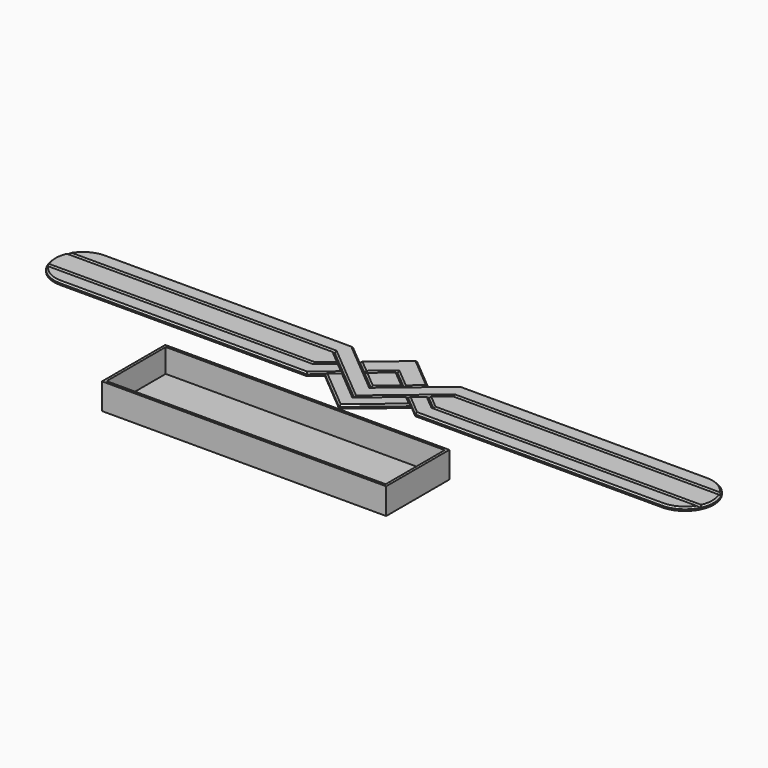
from build123d import *

# Parameters (mm, degrees)
F1_DEPTH  = 2
F3_DEPTH  = 2
F5_DEPTH  = 2
F7_DEPTH  = 2
F9_DEPTH  = 1
F12_DEPTH = 2
F13_SIZE  = 0.99999
F14_W     = 180
F14_H     = 50
F15_DEPTH = 1.6
F16_W     = 180
F16_H     = 50
F16_W_2   = 176.8
F16_H_2   = 46.8
F17_DEPTH = 15


# Not quite as in the source:
# - a fillet or chamfer is up to 0.001 mm smaller than in the source, because OpenCascade refuses the exact size


with BuildPart() as f1:
    # F0 (on Top) → F1 (new body)
    with BuildSketch(Plane.XY):
        Polygon((37.9150851114, 8), (28.3810563706, 0), (37.9150851114, -8), (210, -8), (210, 0), (210, 8), align=None)
    extrude(amount=F1_DEPTH)


with BuildPart() as f1b:
    # F0 (on Top) → F1, piece 2 (new body)
    with BuildSketch(Plane.XY):
        Polygon((-37.9150851114, -8), (-28.3810563706, 0), (-37.9150851114, 8), (-210, 8), (-210, 0), (-210, -8), align=None)
    extrude(amount=F1_DEPTH)


with BuildPart() as f3:
    # F2 (on Top) → F3 (new body)
    with BuildSketch(Plane.XY):
        Polygon((-37.8240925528, 8.25), (0, -23.4881821107), (37.8240925528, 8.25), (210, 8.25), (210, 18.25), (34.1843902102, 18.25), (0, -10.4341092174), (-34.1843902102, 18.25), (-210, 18.25), (-210, 8.25), align=None)
    extrude(amount=F3_DEPTH)


with BuildPart() as f5:
    # F4 (on Top) → F5 (new body)
    with BuildSketch(Plane.XY):
        Polygon((12.4810478052, 0.365085215), (21.6735811226, 8.0785365312), (0, 26.2648304575), (-21.6735811226, 8.0785365312), (-12.4810478052, 0.365085215), (0, 10.8379278251), align=None)
    extrude(amount=F5_DEPTH)


with BuildPart() as f5b:
    # F4 (on Top) → F5, piece 2 (new body)
    with BuildSketch(Plane.XY):
        Polygon((37.8240925528, -8.25), (28.1865908923, -0.1631759112), (20.5261464611, -6.591052008), (34.4207396164, -18.25), (210, -18.25), (210, -8.25), align=None)
    extrude(amount=F5_DEPTH)


with BuildPart() as f5c:
    # F4 (on Top) → F5, piece 3 (new body)
    with BuildSketch(Plane.XY):
        Polygon((-210, -18.25), (-34.4207396164, -18.25), (-20.5261464611, -6.591052008), (-28.1865908923, -0.1631759112), (-37.8240925528, -8.25), (-210, -8.25), align=None)
    extrude(amount=F5_DEPTH)


with BuildPart() as f7:
    # F6 (on Top) → F7 (new body)
    with BuildSketch(Plane.XY):
        Polygon((-27.3324382036, -12.6285607212), (0, -35.563199537), (27.3324382036, -12.6285607212), (20.3316809827, -6.7542279192), (0, -23.814533933), (-20.3316809827, -6.7542279192), align=None)
    extrude(amount=F7_DEPTH)


with BuildPart() as f7b:
    # F6 (on Top) → F7, piece 2 (new body)
    with BuildSketch(Plane.XY):
        Polygon((-12.2865823268, 0.2019093038), (0, -10.107757395), (12.2865823268, 0.2019093038), (0, 10.5115760027), align=None)
    extrude(amount=F7_DEPTH)


with BuildPart() as f9:
    # F8 (on Top) → F9 (new body)
    with BuildSketch(Plane.XY):
        Polygon((21.868046601, 7.9153606201), (0, 26.2648304575), (-21.868046601, 7.9153606201), (-34.1843902102, 18.25), (-210, 18.25), (-210, -18.25), (-34.4207396164, -18.25), (-27.526903682, -12.46538481), (0, -35.563199537), (27.526903682, -12.46538481), (34.4207396164, -18.25), (210, -18.25), (210, 18.25), (34.1843902102, 18.25), align=None)
    extrude(amount=F9_DEPTH)


with BuildPart() as f1_1:
    add(f1.part)

    # F10: union F1b, F3, F5, F5b, F5c, F7, F7b, F9
    add(f1b.part)
    add(f3.part)
    add(f5.part)
    add(f5b.part)
    add(f5c.part)
    add(f7.part)
    add(f7b.part)
    add(f9.part)

    # F11 (on Top) → F12 (cut, through all)
    with BuildSketch(Plane.XY):
        with BuildLine():
            ThreePointArc((190.75, 18.25), (209, 0), (190.75, -18.25))
            Line((190.75, -18.25), (224.6172776222, -18.25))
            Line((224.6172776222, -18.25), (224.6172776222, 18.25))
            Line((224.6172776222, 18.25), (190.75, 18.25))
        make_face()
        with BuildLine():
            Line((-224.6172776222, -18.25), (-190.75, -18.25))
            ThreePointArc((-190.75, -18.25), (-209, 0), (-190.75, 18.25))
            Line((-190.75, 18.25), (-224.6172776222, 18.25))
            Line((-224.6172776222, 18.25), (-224.6172776222, -18.25))
        make_face()
    extrude(amount=F12_DEPTH, mode=Mode.SUBTRACT)

    # F13 (size 1 in the source; OpenCascade refuses exactly that, so slightly less here)
    f13_edges = [f1_1.edges().sort_by_distance(p)[0] for p in [
        (-122.426457, 8.25, 2),
        (-200.302487, 15.550322, 2),
        (-112.467195, 18.25, 2),
        (-17.092195, 3.907945, 2),
        (17.092195, 3.907945, 2),
        (112.467195, 18.25, 2),
        (200.302487, 15.550322, 2),
        (122.426457, 8.25, 2),
        (18.912046, -7.619091, 2),
        (-18.912046, -7.619091, 2),
        (-122.534105, -8, 2),
        (-209, 0, 2),
        (-122.534105, 8, 2),
        (-33.148071, 4, 2),
        (-33.148071, -4, 2),
        (-33.005342, -4.206588, 2),
        (-24.356369, -3.377114, 2),
        (-27.473443, -12.420526, 2),
        (-112.58537, -18.25, 2),
        (-200.302487, -15.550322, 2),
        (-122.426457, -8.25, 2),
        (6.240524, 5.601507, 2),
        (17.077314, 4.221811, 2),
        (10.836791, 17.171683, 2),
        (-10.836791, 17.171683, 2),
        (-17.077314, 4.221811, 2),
        (-6.240524, 5.601507, 2),
        (-6.143291, -4.952924, 2),
        (6.143291, -4.952924, 2),
        (6.143291, 5.356743, 2),
        (-6.143291, 5.356743, 2),
        (-23.83206, -9.691394, 2),
        (-13.666219, -24.09588, 2),
        (13.666219, -24.09588, 2),
        (23.83206, -9.691394, 2),
        (10.16584, -15.284381, 2),
        (-10.16584, -15.284381, 2),
        (122.426457, -8.25, 2),
        (200.302487, -15.550322, 2),
        (112.58537, -18.25, 2),
        (27.473443, -12.420526, 2),
        (24.356369, -3.377114, 2),
        (33.005342, -4.206588, 2),
        (122.534105, 8, 2),
        (209, 0, 2),
        (122.534105, -8, 2),
        (33.148071, -4, 2),
        (33.148071, 4, 2),
    ]]
    chamfer(f13_edges, length=F13_SIZE)


with BuildPart() as f15:
    # F14 (on Top) → F15 (new body)
    with BuildSketch(Plane.XY):
        with Locations((0, -85.7728616616)):
            Rectangle(F14_W, F14_H)
    extrude(amount=F15_DEPTH)

    # F16 (on face) → F17 (join)
    with BuildSketch(Plane.XY.offset(1.6)):
        with Locations((0, -85.7728616616)):
            Rectangle(F16_W, F16_H)
        with Locations((0, -85.7728616616)):
            Rectangle(F16_W_2, F16_H_2, mode=Mode.SUBTRACT)
    extrude(amount=F17_DEPTH)


solid = Compound([f1_1.part, f15.part])
